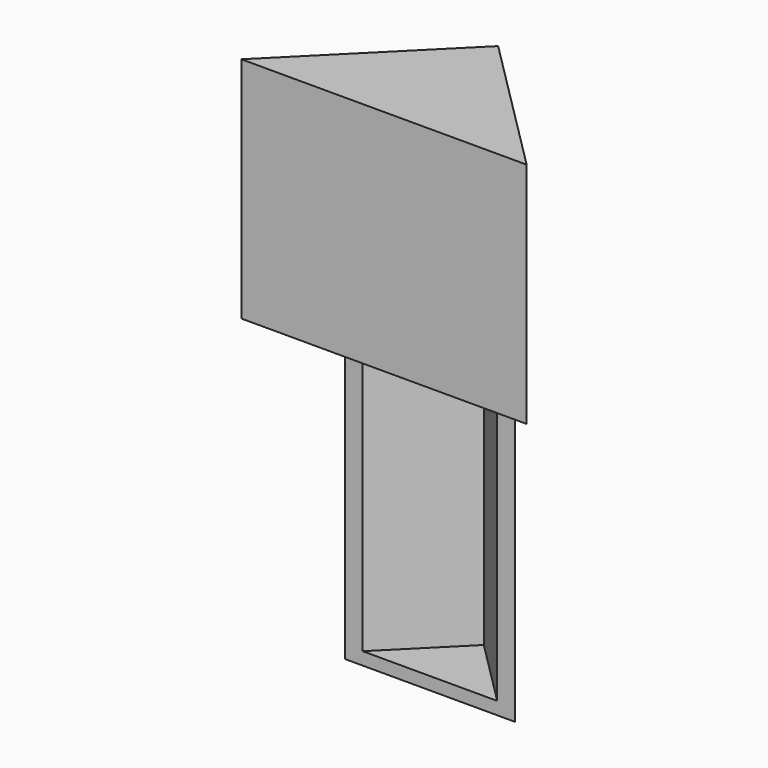
from build123d import *

# Parameters (mm, degrees)
F1_DEPTH = 1219.2
F3_DEPTH = 914.4
F4_T     = 50.8


# Not quite as in the source:
# - a shell that OpenCascade refuses in one call is made with other operations: the cavity is built on its own and cut out


with BuildPart() as f1:
    # F0 (on Top) → F1 (new body)
    with BuildSketch(Plane.XY):
        Polygon((0, 0), (-341.2497326006, -341.2497326006), (341.2497326006, -341.2497326006), align=None)
    extrude(amount=F1_DEPTH)

    # F2 (on face) → F3 (join)
    with BuildSketch(Plane.XY.offset(1219.2)):
        Polygon((341.2497326006, -341.2497326006), (0, 0), (-341.2497326006, -341.2497326006), align=None)
        Polygon((341.2497326006, -341.2497326006), (-341.2497326006, -341.2497326006), (-571.5, -571.5), (571.5, -571.5), align=None)
    extrude(amount=F3_DEPTH)

    # F4: shell of thickness 50.8, made by hand


with BuildPart() as f4_core1:
    # F4_t2: copy of F1
    add(f1.part)

    # the walls: a layer under each face that stays
    f4_faces = [f4_core1.faces().sort_by_distance(p)[0] for p in [
        (-285.75, -285.75, 1066.8),
        (0, -170.6248663003, 0),
        (0, -456.3748663003, 1219.2),
        (0, -571.5, 1676.4),
        (0, -285.75, 2133.6),
        (285.75, -285.75, 1066.8),
    ]]
    thicken(f4_faces, amount=-F4_T, mode=Mode.SUBTRACT)


with BuildPart() as f1_1:
    add(f1.part)

    # what is left inside the walls is the cavity
    f4_cavity = [f4_core1.part.solids().sort_by_distance(p)[0] for p in [
        (-224.069765, -296.630235, 1405.466667),
    ]]
    add(f4_cavity, mode=Mode.SUBTRACT)


solid = f1_1.part
